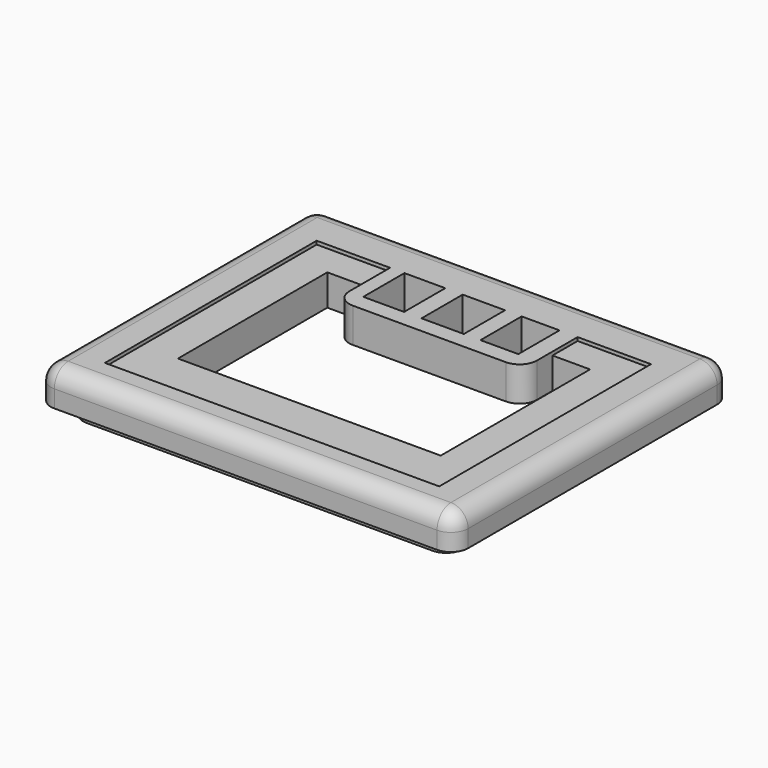
from build123d import *

# Parameters (mm, degrees)
F0_W      = 120.686
F0_H      = 100
F0_W_2    = 76
F0_H_2    = 54
F1_DEPTH  = 10
F3_DEPTH  = 4
F4_R      = 5
F5_W      = 54.2500019073
F5_H      = 10.6249998808
F6_DEPTH  = 10
F8_DEPTH  = 1
F9_W      = 11.812498793
F9_H      = 14.8750022054
F9_W_2    = 12.2500015423
F9_W_3    = 10.9374932945
F10_DEPTH = 25
F11_R     = 5


# Not quite as in the source:
# - a feature names something its author has since deleted; it is built from what else it names


with BuildPart() as f1:
    # F0 (on Top) → F1 (new body)
    with BuildSketch(Plane.XY):
        Rectangle(F0_W, F0_H)
        Rectangle(F0_W_2, F0_H_2, mode=Mode.SUBTRACT)
    extrude(amount=F1_DEPTH)

    # F2 (on face) → F3 (join)
    with BuildSketch(Plane(origin=(0, 0, 0), x_dir=(1, 0, 0), z_dir=(0, 0, -1))):
        with BuildLine():
            ThreePointArc((55, 40), (53.5355339059, 43.5355339059), (50, 45))
            Line((50, 45), (-50, 45))
            ThreePointArc((-50, 45), (-53.5355339059, 43.5355339059), (-55, 40))
            Line((-55, 40), (-55, -40))
            ThreePointArc((-55, -40), (-53.5355339059, -43.5355339059), (-50, -45))
            Line((-50, -45), (50, -45))
            ThreePointArc((50, -45), (53.5355339059, -43.5355339059), (55, -40))
            Line((55, -40), (55, 40))
        make_face()
        with BuildLine():
            Line((-49, 44), (49, 44))
            ThreePointArc((49, 44), (52.5355339059, 42.5355339059), (54, 39))
            Line((54, 39), (54, -39))
            ThreePointArc((54, -39), (52.5355339059, -42.5355339059), (49, -44))
            Line((49, -44), (-49, -44))
            ThreePointArc((-49, -44), (-52.5355339059, -42.5355339059), (-54, -39))
            Line((-54, -39), (-54, 39))
            ThreePointArc((-54, 39), (-52.5355339059, 42.5355339059), (-49, 44))
        make_face(mode=Mode.SUBTRACT)
    extrude(amount=F3_DEPTH)

    # F4
    f4_edges = [f1.edges().sort_by_distance(p)[0] for p in [
        (-60.343, -50, 5),
        (60.343, -50, 5),
        (60.343, 50, 5),
        (-60.343, 50, 5),
        (0, 50, 10),
        (-60.343, 0, 10),
        (0, -50, 10),
        (60.343, 0, 10),
    ]]
    fillet(f4_edges, radius=F4_R)

    # F5 (on face) → F6 (join)
    with BuildSketch(Plane.XY.offset(10)):
        with Locations((0, 21.6875000596)):
            Rectangle(F5_W, F5_H)
    extrude(amount=-F6_DEPTH)

    # F7 (on face) → F8 (cut)
    with BuildSketch(Plane.XY.offset(10)):
        Polygon((48.3437515795, -40.4687528498), (48.3437515795, 36.0937528312), (27.1250009537, 36.0937528312), (27.1250009537, 27), (38, 27), (38, -27), (-38, -27), (-38, 27), (-27.1250009537, 27), (-27.1250009537, 36.0937528312), (-48.3437515795, 36.0937528312), (-48.3437515795, -40.4687528498), align=None)
    extrude(amount=-F8_DEPTH, mode=Mode.SUBTRACT)

    # F9 (on face) → F10 (cut)
    with BuildSketch(Plane.XY.offset(10)):
        with Locations((-17.0625001192, 28.6562517285)):
            Rectangle(F9_W, F9_H)
        with Locations((0, 28.6562517285)):
            Rectangle(F9_W_2, F9_H)
        with Locations((16.4062529802, 28.6562517285)):
            Rectangle(F9_W_3, F9_H)
    extrude(amount=-F10_DEPTH, mode=Mode.SUBTRACT)

    # F11
    f11_edges = [f1.edges().sort_by_distance(p)[0] for p in [
        (-27.125001, 16.375, 5),
        (27.125001, 16.375, 5),
    ]]
    fillet(f11_edges, radius=F11_R)


solid = f1.part
